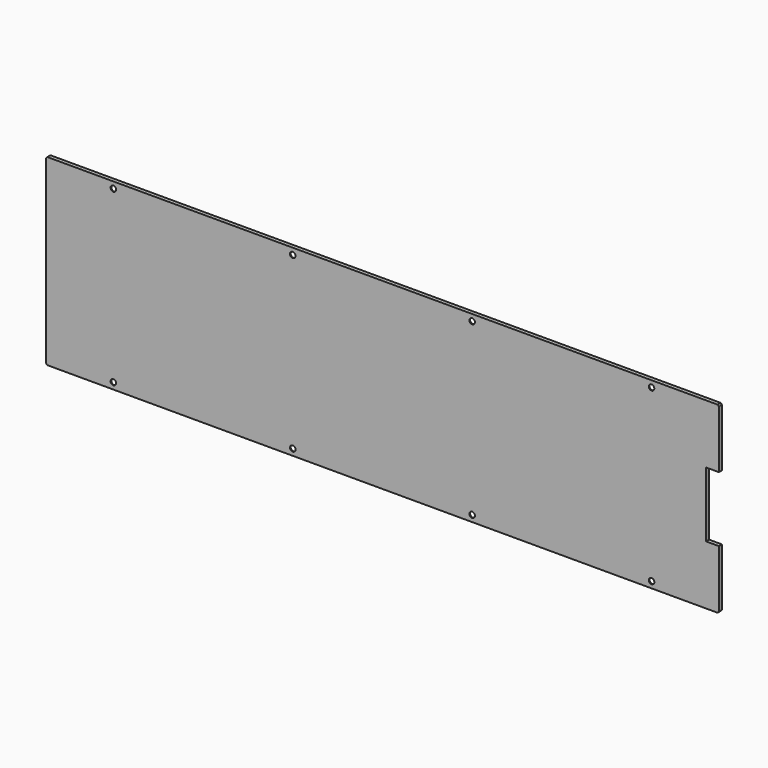
from build123d import *

# Parameters (mm, degrees)
F1_DEPTH       = 3
F3_D           = 4.3
F3_CSINK_D     = 9
F3_CSINK_ANGLE = 90
F4_SIZE        = 1


# Not quite as in the source:
# - a feature names something its author has since deleted; it is built from what else it names


with BuildPart() as f1:
    # F0 (on Front) → F1 (new body)
    with BuildSketch(Plane.XZ):
        Polygon((0, -46.1), (0, 0), (-525, 0), (-525, -143), (0, -143), (0, -96.9), (-10, -96.9), (-10, -46.1), align=None)
    extrude(amount=F1_DEPTH)

    # F3 (through all)
    with Locations(Plane(origin=(0, 0, 0), x_dir=(1, 0, 0), z_dir=(0, 1, 0))):
        with Locations((-472.5, 5), (-332.5, 5), (-192.5, 5), (-52.5, 5), (-52.5, 138), (-192.5, 138), (-332.5, 138), (-472.5, 138)):
            CounterSinkHole(F3_D / 2, F3_CSINK_D / 2, counter_sink_angle=F3_CSINK_ANGLE)

    # F4
    f4_edges = [f1.edges().sort_by_distance(p)[0] for p in [
        (-525, -1.5, 0),
        (-525, -1.5, -143),
        (0, -1.5, -143),
        (0, -1.5, 0),
    ]]
    chamfer(f4_edges, length=F4_SIZE)


solid = f1.part
